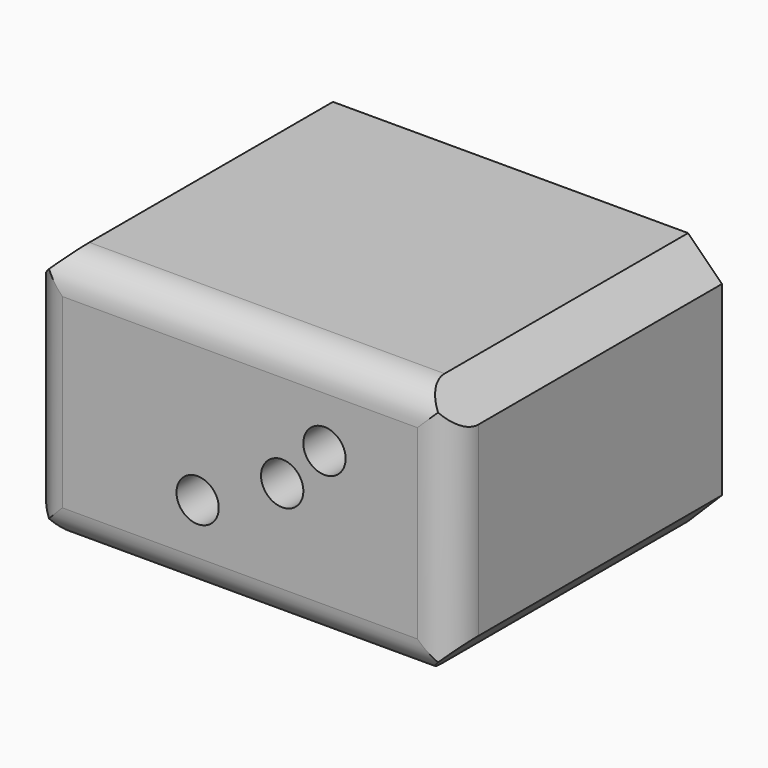
from build123d import *

# Parameters (mm, degrees)
F0_W     = 63.5
F0_H     = 38.1
F1_DEPTH = 50.8
F2_SIZE  = 5.08
F3_R     = 5.08
F3_R_2   = 5.07999
F5_D     = 6.35


# Not quite as in the source:
# - a fillet or chamfer is up to 0.001 mm smaller than in the source, because OpenCascade refuses the exact size


with BuildPart() as f1:
    # F0 (on Front) → F1 (new body)
    with BuildSketch(Plane.XZ):
        with Locations((31.75, 19.05)):
            Rectangle(F0_W, F0_H)
    extrude(amount=-F1_DEPTH)

    # F2
    f2_edges = [f1.edges().sort_by_distance(p)[0] for p in [
        (63.5, 25.4, 38.1),
        (0, 25.4, 38.1),
        (63.5, 25.4, 0),
        (0, 25.4, 0),
    ]]
    chamfer(f2_edges, length=F2_SIZE)

    # F3 (call 1 of 4: OpenCascade refuses the feature's edges together)
    f3_edges = [f1.edges().sort_by_distance(p)[0] for p in [
        (63.5, 0, 19.05),
    ]]
    fillet(f3_edges, radius=F3_R)

    # F3#2 (call 2 of 4)
    f3_2_edges = [f1.edges().sort_by_distance(p)[0] for p in [
        (0, 0, 19.05),
    ]]
    fillet(f3_2_edges, radius=F3_R)

    # F3#3 (call 3 of 4) (radius 5.08 in the source; OpenCascade refuses exactly that, so slightly less here)
    f3_3_edges = [f1.edges().sort_by_distance(p)[0] for p in [
        (31.75, 0, 0),
    ]]
    fillet(f3_3_edges, radius=F3_R_2)

    # F3#4 (call 4 of 4) (radius 5.08 in the source; OpenCascade refuses exactly that, so slightly less here)
    f3_4_edges = [f1.edges().sort_by_distance(p)[0] for p in [
        (31.75, 0, 38.1),
    ]]
    fillet(f3_4_edges, radius=F3_R_2)

    # F5 (through all)
    with Locations(Plane.XZ):
        with Locations((25.4, 12.7), (44.45, 25.4), (38.1, 19.05)):
            Hole(F5_D / 2)


with BuildPart() as f6_1:
    # F6: copy of F1
    add(f1.part.moved(Location((50.8, 50.8, 50.8))))


solid = f1.part
